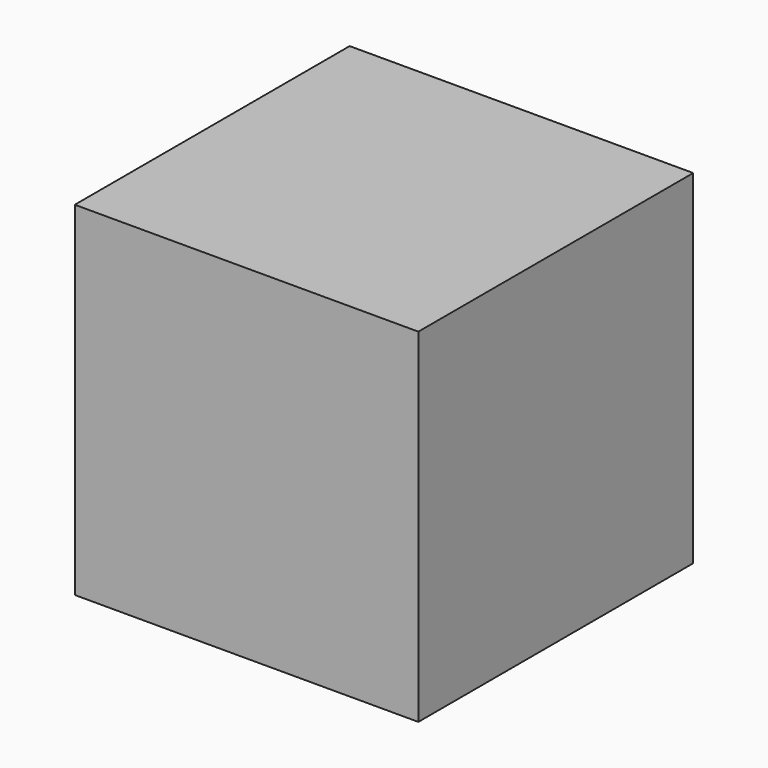
from build123d import *

# Parameters (mm, degrees)
F0_W     = 76.2
F0_H     = 76.2
F1_DEPTH = 38.1
F2_R     = 33.855200569
F3_DEPTH = 172


# Not quite as in the source:
# - an extrude ends at something that could not be found from the text; its depth is read off the source's solid


with BuildPart() as f1:
    # F0 (on Front) → F1 (new body, symmetric)
    with BuildSketch(Plane.XZ):
        with Locations((1.6732892294, 11.20652853)):
            Rectangle(F0_W, F0_H)
    extrude(amount=F1_DEPTH, both=True)

    # F2 (on face) → F3 (cut, through all)
    with BuildSketch(Plane(origin=(-36.4267107706, 0, 0), x_dir=(0, -1, 0), z_dir=(-1, 0, 0))):
        with Locations((0, 14.9851664901)):
            Circle(F2_R)
    extrude(amount=F3_DEPTH, mode=Mode.SUBTRACT)


solid = f1.part
